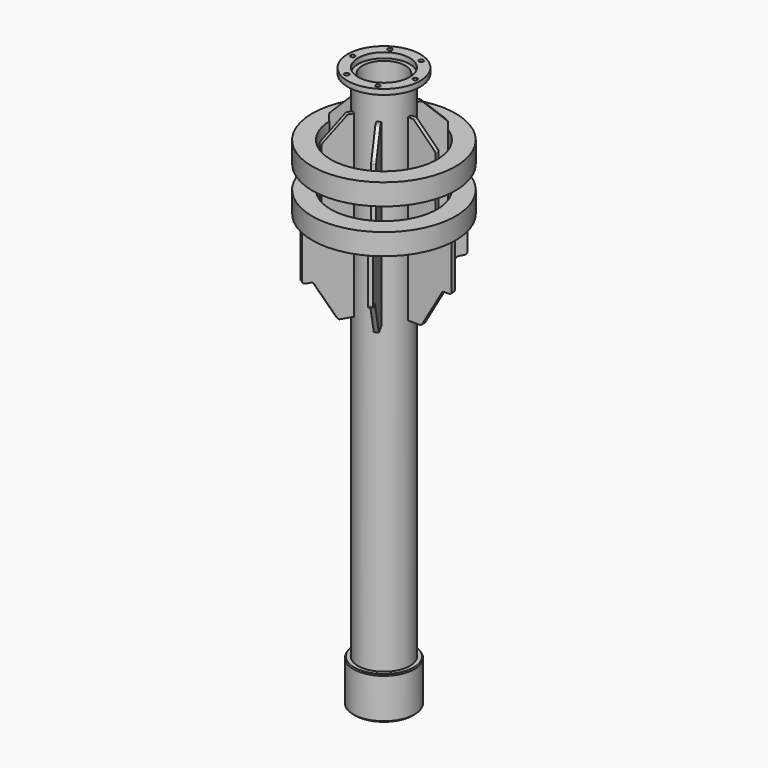
from build123d import *

# Parameters (mm, degrees)
F0_R            = 96.85
F0_R_2          = 80.85
F1_DEPTH        = 1971.5
F2_R            = 136.5
F2_R_2          = 97.25
F3_DEPTH        = 20
F5_D            = 16.5
F5_COPIES_COUNT = 6
F6_W            = 70
F6_H            = 80
F9_DEPTH        = 7.5
F9_COPIES_COUNT = 6
F13_SIZE        = 5


# Not quite as in the source:
# - a fillet or chamfer that OpenCascade refuses, or shapes differently, is made with other operations: its cross-section is extruded or revolved along the edge and cut away or added
# - a pattern or mirror of a feature is missing from the dataset's text; its kind, count and spacing are read off the source's solid


with BuildPart() as f1:
    # F0 (on Top) → F1 (new body)
    with BuildSketch(Plane.XY):
        Circle(F0_R)
        Circle(F0_R_2, mode=Mode.SUBTRACT)
    extrude(amount=-F1_DEPTH)

    # F10 (on Front) → F11 (revolve)
    with BuildSketch(Plane.XZ):
        Polygon((-97.7, -1971.5), (-97.7, -1931.5), (-115, -1931.5), (-115, -2091.5), (-102.25, -2091.5), (-102.25, -2083.5), (-99.75, -2079.1698729811), (-99.75, -1993.8301270189), (-102.25, -1989.5), (-102.25, -1981.5), (-89.35, -1981.5), (-89.35, -1971.5), align=None)
    revolve(axis=Axis((0, 0, 0), (0, 0, 1)))

    # F12: chamfer of 5 x 2.8867513459 on 1 edges, made by hand

    # F12_s1 → F12_t2 (revolve, cut)
    with BuildSketch(Plane.XZ):
        Polygon((-112.1132486541, -1931.5), (-115, -1936.5), (-115, -1931.5), align=None)
    revolve(axis=Axis((0, 0, -1931.5), (0, 0, 1)), mode=Mode.SUBTRACT)

    # F13
    f13_edges = [f1.edges().sort_by_distance(p)[0] for p in [
        (115, 0, -2091.5),
    ]]
    chamfer(f13_edges, length=F13_SIZE)


with BuildPart() as f3:
    # F2 (on face) → F3 (new body)
    with BuildSketch(Plane.XY):
        Circle(F2_R)
        Circle(F2_R_2, mode=Mode.SUBTRACT)
    extrude(amount=F3_DEPTH)

    # F5 (through all)
    with Locations(Plane.XY.offset(20)):
        with Locations((58.75, 101.7579849447)):
            f5 = Hole(F5_D / 2)

    # F5_copies: F5 ×6 about axis
    f5_copies_axis = Axis((0, 0, 0), (0, 0, 1))
    for i in range(1, F5_COPIES_COUNT):
        add(f5.rotate(f5_copies_axis, i * 360 / F5_COPIES_COUNT), mode=Mode.SUBTRACT)


with BuildPart() as f7:
    # F6 (on Front) → F7 (revolve)
    with BuildSketch(Plane.XZ):
        with Locations((-235, -260)):
            Rectangle(F6_W, F6_H)
    revolve(axis=Axis((0, 0, 0), (0, 0, 1)))


with BuildPart() as f7b:
    # F6 (on Front) → F7, piece 2 (revolve)
    with BuildSketch(Plane.XZ):
        with Locations((-235, -425)):
            Rectangle(F6_W, F6_H)
    revolve(axis=Axis((0, 0, 0), (0, 0, 1)))


with BuildPart() as f9:
    # F8 (on Front) → F9 (new body, symmetric)
    with BuildSketch(Plane.XZ):
        with BuildLine():
            Line((-96.85, -783.8140646055), (-96.85, -109.8140646055))
            Line((-96.85, -109.8140646055), (-112.7078643763, -109.8140646055))
            ThreePointArc((-112.7078643763, -109.8140646055), (-116.5346986999, -110.5752692804), (-119.7789321881, -112.7429967936))
            Line((-119.7789321881, -112.7429967936), (-197.0710678119, -190.0351324174))
            ThreePointArc((-197.0710678119, -190.0351324174), (-199.2387953251, -193.2793659056), (-200, -197.1062002292))
            Line((-200, -197.1062002292), (-200, -465))
            Line((-200, -465), (-260.85, -465))
            Line((-260.85, -465), (-260.85, -635.25))
            ThreePointArc((-260.85, -635.25), (-257.9210678119, -642.3210678119), (-250.85, -645.25))
            Line((-250.85, -645.25), (-232.6235026919, -645.25))
            ThreePointArc((-232.6235026919, -645.25), (-227.6235026919, -646.5897459622), (-223.9632486541, -650.25))
            Line((-223.9632486541, -650.25), (-149.7367513459, -778.8140646055))
            ThreePointArc((-149.7367513459, -778.8140646055), (-146.0764973081, -782.4743186434), (-141.0764973081, -783.8140646055))
            Line((-141.0764973081, -783.8140646055), (-96.85, -783.8140646055))
        make_face()
    extrude(amount=F9_DEPTH, both=True)


with BuildPart() as f9_copies_1:
    # F9_copies: instance of F9
    add(f9.part.rotate(Axis((0, 0, 0), (0, 0, 1)), 1 * 360 / F9_COPIES_COUNT))


with BuildPart() as f9_copies_2:
    # F9_copies: instance of F9
    add(f9.part.rotate(Axis((0, 0, 0), (0, 0, 1)), 2 * 360 / F9_COPIES_COUNT))


with BuildPart() as f9_copies_3:
    # F9_copies: instance of F9
    add(f9.part.rotate(Axis((0, 0, 0), (0, 0, 1)), 3 * 360 / F9_COPIES_COUNT))


with BuildPart() as f9_copies_4:
    # F9_copies: instance of F9
    add(f9.part.rotate(Axis((0, 0, 0), (0, 0, 1)), 4 * 360 / F9_COPIES_COUNT))


with BuildPart() as f9_copies_5:
    # F9_copies: instance of F9
    add(f9.part.rotate(Axis((0, 0, 0), (0, 0, 1)), 5 * 360 / F9_COPIES_COUNT))


solid = Compound([f1.part, f3.part, f7.part, f7b.part, f9.part, f9_copies_1.part, f9_copies_2.part, f9_copies_3.part, f9_copies_4.part, f9_copies_5.part])
